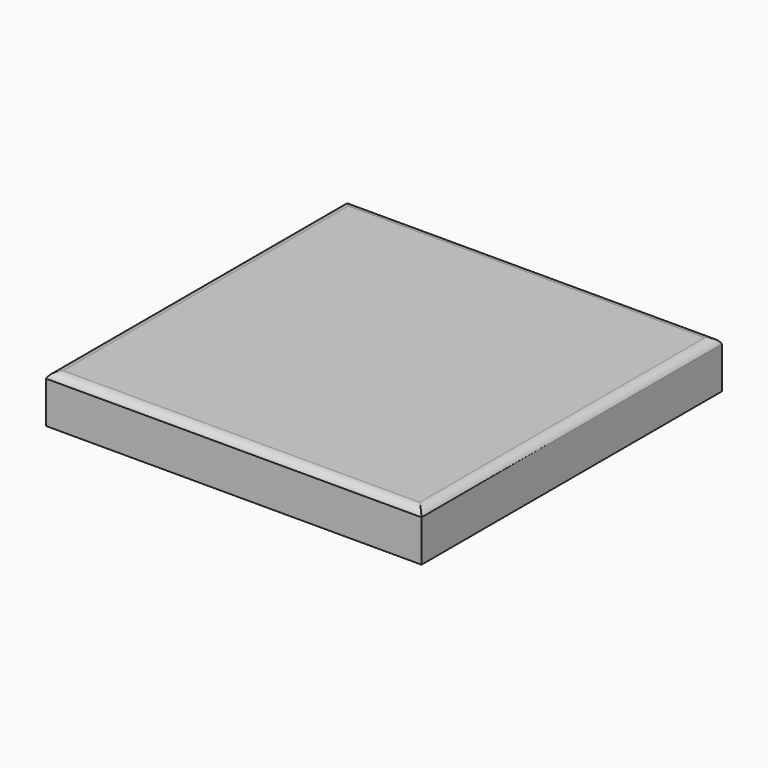
from build123d import *

# Parameters (mm, degrees)
F0_W        = 180
F0_H        = 180
F1_DEPTH    = 3
F3_DEPTH    = 20
F4_DEPTH    = 20
F5_DEPTH    = 20
F6_DEPTH    = 20
F7_T1_DEPTH = 202.9128784748
F7_T3_DEPTH = 202.9128784748


# Not quite as in the source:
# - a fillet or chamfer that OpenCascade refuses, or shapes differently, is made with other operations: its cross-section is extruded or revolved along the edge and cut away or added


with BuildPart() as f1:
    # F0 (on Top) → F1 (new body)
    with BuildSketch(Plane.XY):
        with Locations((90, -90)):
            Rectangle(F0_W, F0_H)
    extrude(amount=-F1_DEPTH)

    # F7: fillet of radius 5 on 4 edges, made by hand

    # F7_s2 → F7_t1 (cut)
    with BuildSketch(Plane.YZ.offset(-11.4564392374)):
        with BuildLine():
            ThreePointArc((-180, -3), (-178.1560370926, -0.8166998673), (-175.417424305, 0))
            Line((-175.417424305, 0), (-180, 0))
            Line((-180, 0), (-180, -3))
        make_face()
        with BuildLine():
            ThreePointArc((0, -3), (-1.8439629074, -0.8166998673), (-4.582575695, 0))
            Line((-4.582575695, 0), (0, 0))
            Line((0, 0), (0, -3))
        make_face()
    extrude(amount=F7_T1_DEPTH, mode=Mode.SUBTRACT)

    # F7_s4 → F7_t3 (cut)
    with BuildSketch(Plane.XZ.offset(-11.4564392374)):
        with BuildLine():
            ThreePointArc((180, -3), (178.1560370926, -0.8166998673), (175.417424305, 0))
            Line((175.417424305, 0), (180, 0))
            Line((180, 0), (180, -3))
        make_face()
        with BuildLine():
            ThreePointArc((0, -3), (1.8439629074, -0.8166998673), (4.582575695, 0))
            Line((4.582575695, 0), (0, 0))
            Line((0, 0), (0, -3))
        make_face()
    extrude(amount=F7_T3_DEPTH, mode=Mode.SUBTRACT)


with BuildPart() as f3:
    # F2 (on face) → F3 (new body)
    with BuildSketch(Plane(origin=(0, 0, -3), x_dir=(1, 0, 0), z_dir=(0, 0, -1))):
        Polygon((0, 180), (8, 172), (172, 172), (180, 180), align=None)
    extrude(amount=F3_DEPTH)


with BuildPart() as f4:
    # F2 (on face) → F4 (new body, through all)
    with BuildSketch(Plane(origin=(0, 0, -3), x_dir=(1, 0, 0), z_dir=(0, 0, -1))):
        Polygon((8, 8), (8, 172), (0, 180), (0, 0), align=None)
    extrude(amount=F4_DEPTH)


with BuildPart() as f5:
    # F2 (on face) → F5 (new body, through all)
    with BuildSketch(Plane(origin=(0, 0, -3), x_dir=(1, 0, 0), z_dir=(0, 0, -1))):
        Polygon((180, 180), (172, 172), (172, 8), (180, 0), align=None)
    extrude(amount=F5_DEPTH)


with BuildPart() as f6:
    # F2 (on face) → F6 (new body, through all)
    with BuildSketch(Plane(origin=(0, 0, -3), x_dir=(1, 0, 0), z_dir=(0, 0, -1))):
        Polygon((172, 8), (8, 8), (0, 0), (180, 0), align=None)
    extrude(amount=F6_DEPTH)


solid = Compound([f1.part, f3.part, f4.part, f5.part, f6.part])
